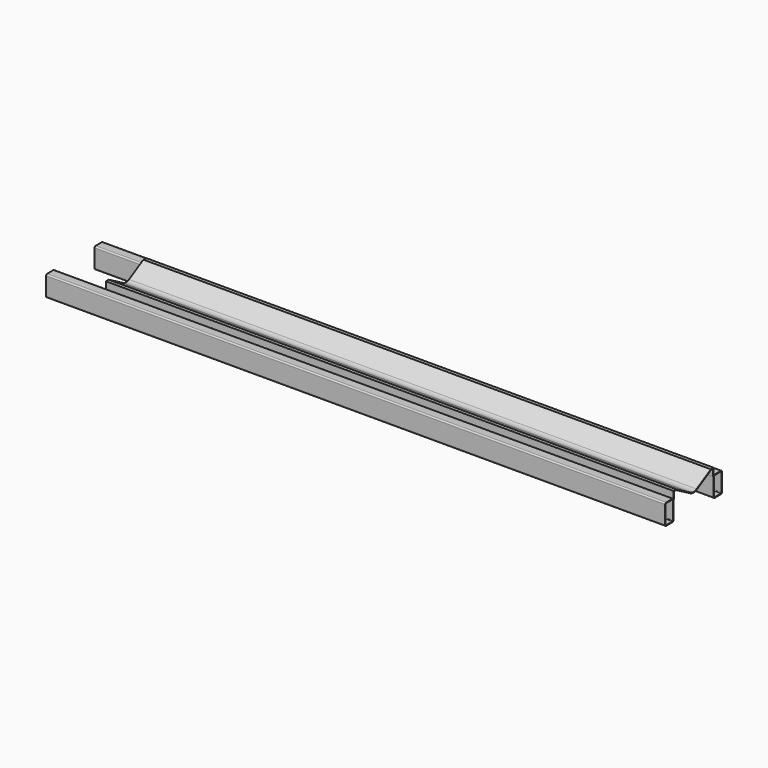
from build123d import *

# Parameters (mm, degrees)
F1_DEPTH = 6096
F2_DEPTH = 5588


# Not quite as in the source:
# - a feature names something its author has since deleted; it is built from what else it names


with BuildPart() as f1:
    # F0 (on Right) → F1 (new body)
    with BuildSketch(Plane.YZ):
        with BuildLine():
            Line((-278.751844046, 57.15), (-336.55, 57.15))
            ThreePointArc((-336.55, 57.15), (-345.5302561211, 53.4302561211), (-349.25, 44.45))
            Line((-349.25, 44.45), (-349.25, -133.35))
            ThreePointArc((-349.25, -133.35), (-345.5302561211, -142.3302561211), (-336.55, -146.05))
            Line((-336.55, -146.05), (-260.35, -146.05))
            ThreePointArc((-260.35, -146.05), (-251.3697438789, -142.3302561211), (-247.65, -133.35))
            Line((-247.65, -133.35), (-247.65, 44.45))
            ThreePointArc((-247.65, 44.45), (-251.3697438789, 53.4302561211), (-260.35, 57.15))
            Line((-260.35, 57.15), (-268.1402802436, 57.15))
            Line((-268.1402802436, 57.15), (-269.3472818438, 57.15))
            Line((-269.3472818438, 57.15), (-278.751844046, 57.15))
        make_face()
        with BuildLine():
            ThreePointArc((-342.9, 44.45), (-341.0401280605, 48.9401280605), (-336.55, 50.8))
            Line((-336.55, 50.8), (-260.35, 50.8))
            ThreePointArc((-260.35, 50.8), (-255.8598719395, 48.9401280605), (-254, 44.45))
            Line((-254, 44.45), (-254, -133.35))
            ThreePointArc((-254, -133.35), (-255.8598719395, -137.8401280605), (-260.35, -139.7))
            Line((-260.35, -139.7), (-336.55, -139.7))
            ThreePointArc((-336.55, -139.7), (-341.0401280605, -137.8401280605), (-342.9, -133.35))
            Line((-342.9, -133.35), (-342.9, 44.45))
        make_face(mode=Mode.SUBTRACT)
    extrude(amount=-F1_DEPTH)


with BuildPart() as f1b:
    # F0 (on Right) → F1, piece 2 (new body)
    with BuildSketch(Plane.YZ):
        with BuildLine():
            ThreePointArc((260.35, 57.15), (251.3697438789, 53.4302561211), (247.65, 44.45))
            Line((247.65, 44.45), (247.65, -133.35))
            ThreePointArc((247.65, -133.35), (251.3697438789, -142.3302561211), (260.35, -146.05))
            Line((260.35, -146.05), (336.55, -146.05))
            ThreePointArc((336.55, -146.05), (345.5302561211, -142.3302561211), (349.25, -133.35))
            Line((349.25, -133.35), (349.25, 44.45))
            ThreePointArc((349.25, 44.45), (345.5302561211, 53.4302561211), (336.55, 57.15))
            Line((336.55, 57.15), (260.35, 57.15))
        make_face()
        with BuildLine():
            Line((260.35, 50.8), (336.55, 50.8))
            ThreePointArc((336.55, 50.8), (341.0401280605, 48.9401280605), (342.9, 44.45))
            Line((342.9, 44.45), (342.9, -133.35))
            ThreePointArc((342.9, -133.35), (341.0401280605, -137.8401280605), (336.55, -139.7))
            Line((336.55, -139.7), (260.35, -139.7))
            ThreePointArc((260.35, -139.7), (255.8598719395, -137.8401280605), (254, -133.35))
            Line((254, -133.35), (254, 44.45))
            ThreePointArc((254, 44.45), (255.8598719395, 48.9401280605), (260.35, 50.8))
        make_face(mode=Mode.SUBTRACT)
    extrude(amount=-F1_DEPTH)


with BuildPart() as f2:
    # F0 (on Right) → F2 (new body)
    with BuildSketch(Plane.YZ):
        with BuildLine():
            Line((-247.65, 120.65), (-247.65, 44.45))
            Line((-247.65, 44.45), (-241.3, 44.45))
            Line((-241.3, 44.45), (-241.3, 114.3))
            Line((-241.3, 114.3), (-214.7923633436, 114.3))
            Line((-214.7923633436, 114.3), (-40.6681247176, 15.7258547021))
            ThreePointArc((-40.6681247176, 15.7258547021), (0, 5.0132135897), (40.6681247176, 15.7258547021))
            Line((40.6681247176, 15.7258547021), (214.7923633436, 114.3))
            Line((214.7923633436, 114.3), (241.3, 114.3))
            Line((241.3, 114.3), (241.3, 44.45))
            Line((241.3, 44.45), (247.65, 44.45))
            Line((247.65, 44.45), (247.65, 120.65))
            Line((247.65, 120.65), (213.1196707487, 120.65))
            Line((213.1196707487, 120.65), (37.5398074317, 21.2518053858))
            ThreePointArc((37.5398074317, 21.2518053858), (0, 11.3632135897), (-37.5398074317, 21.2518053858))
            Line((-37.5398074317, 21.2518053858), (-213.1196707487, 120.65))
            Line((-213.1196707487, 120.65), (-247.65, 120.65))
        make_face()
    extrude(amount=-F2_DEPTH)


solid = Compound([f1.part, f1b.part, f2.part])
